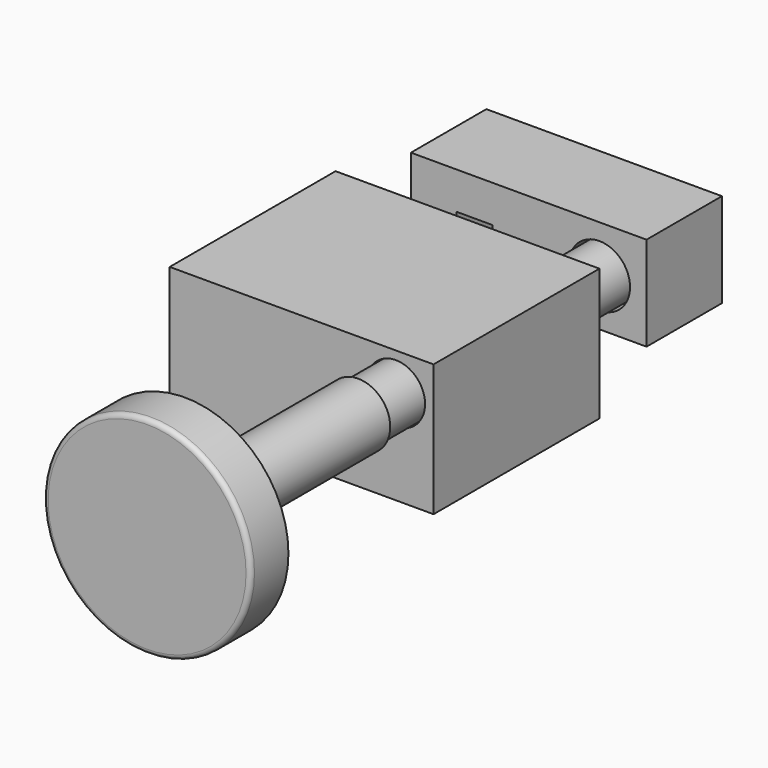
from build123d import *

# Parameters (mm, degrees)
F0_W      = 28
F0_H      = 4.3
F0_H_2    = 9.7
F0_W_2    = 13.5
F0_H_3    = 7.7
F0_R      = 3.1
F1_DEPTH  = 22
F2_W      = 13.5
F2_H      = 7.7
F3_DEPTH  = 8
F4_R      = 1.3
F5_DEPTH  = 12
F8_R      = 11
F9_DEPTH  = 5
F10_R     = 3
F11_DEPTH = 55
F12_W     = 25
F12_H     = 10
F13_DEPTH = 10
F14_W     = 3.8
F14_H     = 3.8
F15_DEPTH = 7
F14_R     = 3.25
F16_DEPTH = 8.5
F17_R     = 3.4
F18_DEPTH = 23
F19_R     = 3
F20_DEPTH = 7.5
F21_R     = 1.3
F22_DEPTH = 12
F23_R     = 1.6
F24_DEPTH = 25
F25_R     = 0.5


with BuildPart() as f1:
    # F0 (on Front) → F1 (new body)
    with BuildSketch(Plane.XZ):
        with Locations((-36, -7)):
            Rectangle(F0_W, F0_H)
        with Locations((-36, 0)):
            Rectangle(F0_W, F0_H_2)
        with Locations((-41.75, 0)):
            Rectangle(F0_W_2, F0_H_3, mode=Mode.SUBTRACT)
        with Locations((-26, 0.85)):
            Circle(F0_R, mode=Mode.SUBTRACT)
    extrude(amount=-F1_DEPTH)

    # F2 (on face) → F3 (join)
    with BuildSketch(Plane.XZ):
        with Locations((-41.75, 0)):
            Rectangle(F2_W, F2_H)
    extrude(amount=-F3_DEPTH)

    # F4 (on face) → F5 (cut)
    with BuildSketch(Plane(origin=(0, 0, -9.15), x_dir=(1, 0, 0), z_dir=(0, 0, -1))):
        with Locations((-32, -3.5)):
            Circle(F4_R)
        with Locations((-32, -18.5)):
            Circle(F4_R)
    extrude(amount=-F5_DEPTH, mode=Mode.SUBTRACT)


with BuildPart() as f9:
    # F8 (on offset) → F9 (new body)
    with BuildSketch(Plane.XZ.offset(28)):
        with Locations((-26, 0.85)):
            Circle(F8_R)
    extrude(amount=F9_DEPTH)

    # F10 (on face) → F11 (join)
    with BuildSketch(Plane(origin=(0, -28, 0), x_dir=(-1, 0, 0), z_dir=(0, 1, 0))):
        with Locations((26, 0.85)):
            Circle(F10_R)
    extrude(amount=F11_DEPTH)

    # F17 (on face) → F18 (join)
    with BuildSketch(Plane.XZ.offset(28)):
        with Locations((-26, 0.85)):
            Circle(F17_R)
    extrude(amount=-F18_DEPTH)

    # F19 (on face) → F20 (join)
    with BuildSketch(Plane(origin=(0, 27, 0), x_dir=(-1, 0, 0), z_dir=(0, 1, 0))):
        with Locations((26, 0.85)):
            Circle(F19_R)
    extrude(amount=F20_DEPTH)

    # F21 (on face) → F22 (cut)
    with BuildSketch(Plane(origin=(0, 34.5, 0), x_dir=(-1, 0, 0), z_dir=(0, 1, 0))):
        with Locations((26, 0.85)):
            Circle(F21_R)
    extrude(amount=-F22_DEPTH, mode=Mode.SUBTRACT)

    # F25
    f25_edges = [f9.edges().sort_by_distance(p)[0] for p in [
        (-37, -33, 0.85),
    ]]
    fillet(f25_edges, radius=F25_R)


with BuildPart() as f13:
    # F12 (on offset) → F13 (new body)
    with BuildSketch(Plane(origin=(0, 27, 0), x_dir=(-1, 0, 0), z_dir=(0, 1, 0))):
        with Locations((33.5, 0.85)):
            Rectangle(F12_W, F12_H)
    extrude(amount=F13_DEPTH)

    # F14 (on face) → F15 (cut)
    with BuildSketch(Plane.XZ.offset(-27)):
        with Locations((-39.25, 0)):
            Rectangle(F14_W, F14_H)
    extrude(amount=-F15_DEPTH, mode=Mode.SUBTRACT)

    # F14 (on face) → F16 (cut)
    with BuildSketch(Plane.XZ.offset(-27)):
        with Locations((-26, 0.85)):
            Circle(F14_R)
    extrude(amount=-F16_DEPTH, mode=Mode.SUBTRACT)

    # F23 (on face) → F24 (cut)
    with BuildSketch(Plane(origin=(0, 37, 0), x_dir=(-1, 0, 0), z_dir=(0, 1, 0))):
        with Locations((26, 0.85)):
            Circle(F23_R)
    extrude(amount=-F24_DEPTH, mode=Mode.SUBTRACT)


solid = Compound([f1.part, f9.part, f13.part])
